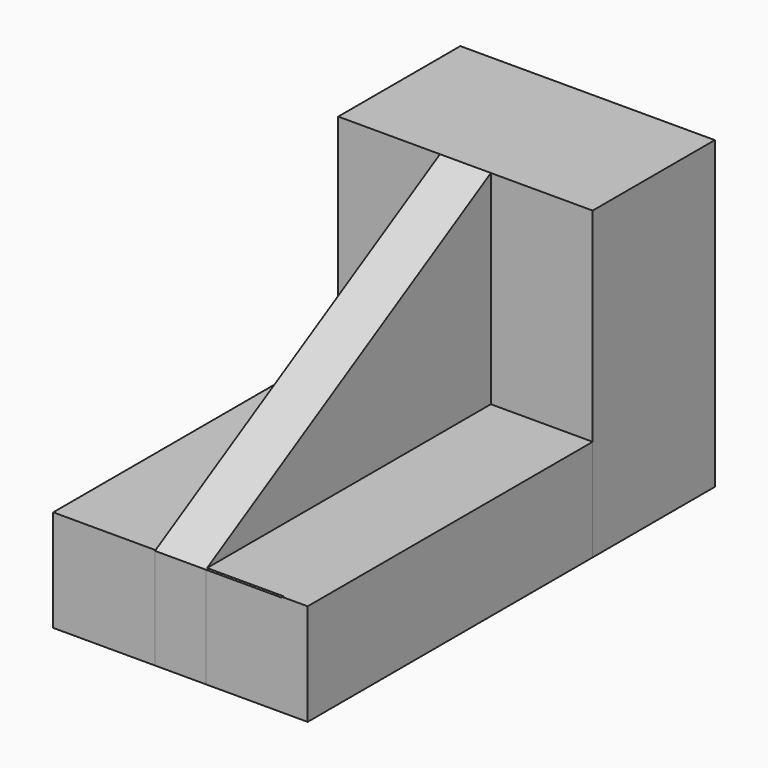
from build123d import *

# Parameters (mm, degrees)
F0_W     = 20
F0_H     = 70
F1_DEPTH = 20
F2_DEPTH = 60
F3_DEPTH = 60
F5_DEPTH = 25
F6_W     = 30
F6_H     = 10
F7_DEPTH = 107


with BuildPart() as f1:
    # F0 (on Top) → F1 (new body)
    with BuildSketch(Plane.XY):
        with Locations((-10, 2.2590903938)):
            Rectangle(F0_W, F0_H)
    extrude(amount=F1_DEPTH)

    # F6 (on face) → F7 (cut)
    with BuildSketch(Plane(origin=(-20, 0, 0), x_dir=(0, -1, 0), z_dir=(-1, 0, 0))):
        with Locations((-2.2590903938, 5)):
            Rectangle(F6_W, F6_H)
        Polygon((-27.2590903938, 10), (-17.2590903938, 0), (-17.2590903938, 10), align=None)
        Polygon((12.7409096062, 10), (12.7409096062, 0), (22.7409096062, 10), align=None)
    extrude(amount=-F7_DEPTH, mode=Mode.SUBTRACT)


with BuildPart() as f1b:
    # F0 (on Top) → F1, piece 2 (new body)
    with BuildSketch(Plane.XY):
        with Locations((20, 2.2590903938)):
            Rectangle(F0_W, F0_H)
    extrude(amount=F1_DEPTH)


with BuildPart() as f2:
    # F0 (on Top) → F2 (new body)
    with BuildSketch(Plane.XY):
        Polygon((30, 67.2590903938), (-20, 67.2590903938), (-20, 37.2590903938), (0, 37.2590903938), (5, 37.2590903938), (10, 37.2590903938), (30, 37.2590903938), align=None)
    extrude(amount=F2_DEPTH)


with BuildPart() as f3:
    # F0 (on Top) → F3 (new body)
    with BuildSketch(Plane.XY):
        Polygon((5, 37.2590903938), (0, 37.2590903938), (0, -32.7409096062), (10, -32.7409096062), (10, 37.2590903938), align=None)
    extrude(amount=F3_DEPTH)


with BuildPart() as f5_tool:
    # F4 (on face) → F5 (new body)
    with BuildSketch(Plane(origin=(0, 0, 0), x_dir=(0, -1, 0), z_dir=(-1, 0, 0))):
        Polygon((32.7409096062, 60), (-37.2590903938, 60), (32.7409096062, 19.8320876807), align=None)
    extrude(amount=-F5_DEPTH)


with BuildPart() as f1b_1:
    add(f1b.part)

    # F5: cut by f5_tool
    add(f5_tool.part, mode=Mode.SUBTRACT)


with BuildPart() as f3_1:
    add(f3.part)

    # F5: cut by f5_tool
    add(f5_tool.part, mode=Mode.SUBTRACT)


solid = Compound([f1.part, f2.part, f1b_1.part, f3_1.part])
